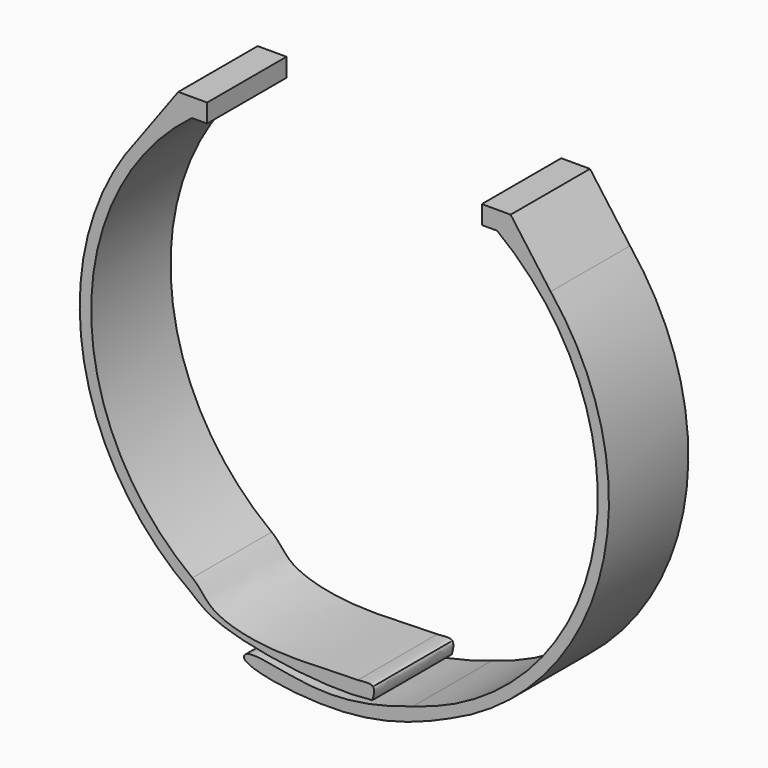
from build123d import *

# Parameters (mm, degrees)
F1_DEPTH = 13
F2_W     = 1
F2_H     = 1
F3_DEPTH = 1
F4_W     = 1
F4_H     = 1
F5_DEPTH = 1


with BuildPart() as f1:
    # F0 (on Front) → F1 (new body)
    with BuildSketch(Plane.XZ):
        with BuildLine():
            Line((-20.6169642951, 29.1691173466), (-25.8707289793, 21.9952982577))
            ThreePointArc((-25.8707289793, 21.9952982577), (-33.1953355355, -4.5741350256), (-18.8384999186, -28.0999913812))
            add(Edge.make_bspline(
                [(4.8171508045, -32.7365776711), (3.7167628648, -32.8648680628), (-2.0078676806, -33.2386642036), (-15.1145375012, -31.2964158038), (-17.8746474637, -28.9047208245), (-18.8384999186, -28.0999913812)],
                knots=[0.2111724842, 0.2111724842, 0.2111724842, 0.2111724842, 0.3278897204, 0.7679049251, 1, 1, 1, 1], degree=3))
            add(Edge.make_bspline(
                [(4.8171508045, -32.7365776711), (4.989720658, -32.1658326051), (5.1633975969, -31.4424290663), (4.8911119625, -31.138586367)],
                knots=[0, 0, 0, 0, 0.4730600729, 0.4730600729, 0.4730600729, 0.4730600729], degree=3))
            add(Edge.make_bspline(
                [(2.9094921994, -31.025311802), (3.6349605155, -31.0329879922), (4.3019062728, -31.0657304896), (4.8911119625, -31.138586367)],
                knots=[0.7618465854, 0.7618465854, 0.7618465854, 0.7618465854, 0.8320559926, 0.8320559926, 0.8320559926, 0.8320559926], degree=3))
            add(Edge.make_bspline(
                [(-18.777262778, -26.2892581576), (-17.690403063, -27.0949326256), (-16.5513786536, -29.8310253675), (-7.5403271997, -31.7066149297), (0.1554117452, -30.9961708391), (2.9094921994, -31.025311802)],
                knots=[0, 0, 0, 0, 0.1916771355, 0.4953120559, 0.7618465854, 0.7618465854, 0.7618465854, 0.7618465854], degree=3))
            ThreePointArc((-18.777262778, -26.2892581576), (-32.0321750084, 0.2104453607), (-18.8384999186, 26.7406907877))
            Line((-18.8384999186, 26.7406907877), (-18.8384999186, 27.7406907877))
            Line((-18.8384999186, 27.7406907877), (-17.8384999186, 27.7406907877))
            Line((-17.8384999186, 27.7406907877), (-17.8384999186, 26.7406907877))
            Line((-17.8384999186, 26.7406907877), (-16.8384999186, 26.7406907877))
            Line((-16.8384999186, 26.7406907877), (-16.8384999186, 29.1691173466))
            Line((-16.8384999186, 29.1691173466), (-20.6169642951, 29.1691173466))
        make_face()
        with BuildLine():
            add(Edge.make_bspline(
                [(2.9094921994, -31.025311802), (3.6349605155, -31.0329879922), (4.3019062728, -31.0657304896), (4.8911119625, -31.138586367)],
                knots=[0.7618465854, 0.7618465854, 0.7618465854, 0.7618465854, 0.8320559926, 0.8320559926, 0.8320559926, 0.8320559926], degree=3))
            add(Edge.make_bspline(
                [(4.8911119625, -31.138586367), (4.5878139659, -30.8001370686), (3.7311811009, -30.9822642844), (2.9094921994, -31.025311802)],
                knots=[0.4730600729, 0.4730600729, 0.4730600729, 0.4730600729, 1, 1, 1, 1], degree=3))
        make_face()
    extrude(amount=F1_DEPTH)

    # F2 (on face) → F3 (join)
    with BuildSketch(Plane(origin=(0, 0, 27.7406907877), x_dir=(1, 0, 0), z_dir=(0, 0, -1))):
        with Locations((-18.3384999186, 12.5)):
            Rectangle(F2_W, F2_H)
        with Locations((-18.3384999186, 0.5)):
            Rectangle(F2_W, F2_H)
    extrude(amount=F3_DEPTH)


with BuildPart() as f1b:
    # F0 (on Front) → F1, piece 2 (new body)
    with BuildSketch(Plane.XZ):
        with BuildLine():
            ThreePointArc((21.1615000814, 26.7406907877), (33.7800460803, -5.9036210065), (10.1370342304, -31.7084032437))
            add(Edge.make_bspline(
                [(10.1370342304, -31.7084032437), (8.1415153454, -32.4297144445), (2.6951474398, -33.9763337281), (-4.5691980179, -33.9053878557), (-11.480754016, -32.0767755357), (-12.8163446055, -34.2765928251), (2.3457925371, -36.6938021282), (11.155715078, -33.293928505), (15.0117562615, -31.5189600018)],
                knots=[0, 0, 0, 0, 0.1663185786, 0.339043873, 0.4942349507, 0.5478616611, 0.7663253639, 1, 1, 1, 1], degree=3))
            ThreePointArc((15.0117562615, -31.5189600018), (34.814276549, -8.0142387453), (28.1780562432, 21.9952982577))
            Line((28.1780562432, 21.9952982577), (22.9360007514, 29.1691173466))
            Line((22.9360007514, 29.1691173466), (19.1615000814, 29.1691173466))
            Line((19.1615000814, 29.1691173466), (19.1615000814, 26.7406907877))
            Line((19.1615000814, 26.7406907877), (20.1615000814, 26.7406907877))
            Line((20.1615000814, 26.7406907877), (20.1615000814, 27.7406907877))
            Line((20.1615000814, 27.7406907877), (21.1615000814, 27.7406907877))
            Line((21.1615000814, 27.7406907877), (21.1615000814, 26.7406907877))
        make_face()
    extrude(amount=F1_DEPTH)

    # F4 (on face) → F5 (join)
    with BuildSketch(Plane(origin=(0, 0, 27.7406907877), x_dir=(1, 0, 0), z_dir=(0, 0, -1))):
        with Locations((20.6615000814, 0.5)):
            Rectangle(F4_W, F4_H)
        with Locations((20.6615000814, 12.5)):
            Rectangle(F4_W, F4_H)
    extrude(amount=F5_DEPTH)


solid = Compound([f1.part, f1b.part])
